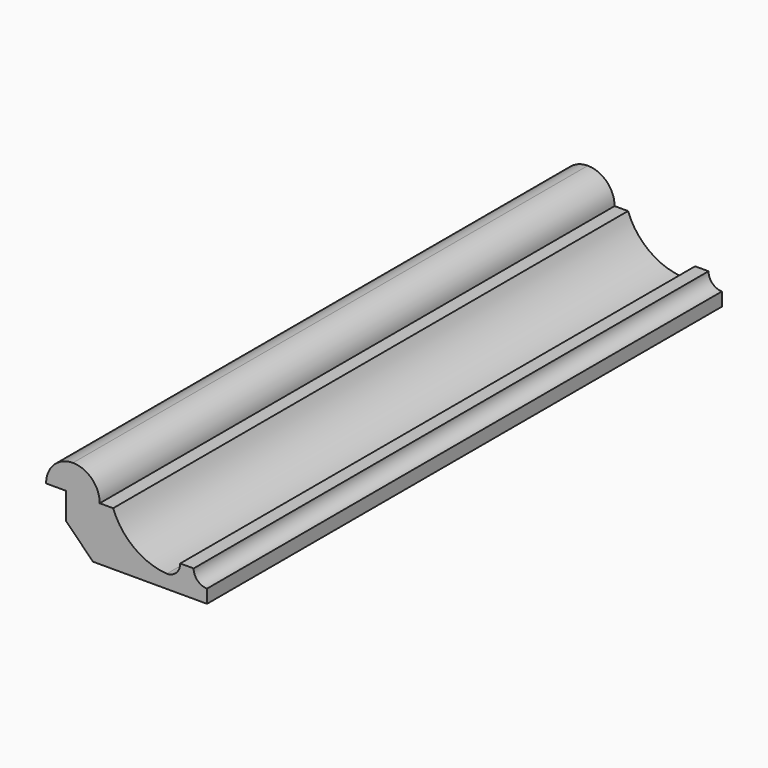
from build123d import *

# Parameters (mm, degrees)
F1_DEPTH = 152.4


# Not quite as in the source:
# - ends of sketch curves that miss each other by under 0.0002 mm in the source are joined


with BuildPart() as f1:
    # F0 (on Front) → F1 (new body)
    with BuildSketch(Plane.XZ):
        with BuildLine():
            ThreePointArc((-6.352921, 3.1764732), (-8.2136484806, 7.6686667194), (-12.705842, 9.5293942))
            ThreePointArc((-12.705842, 9.5293942), (-17.1980355194, 7.6686667194), (-19.058763, 3.1764732))
            Line((-19.058763, 3.1764732), (-14.2940786, 3.1764732))
            Line((-14.2940786, 3.1764732), (-14.2940786, -3.1764478))
            Line((-14.2940786, -3.1764478), (-7.9411576, -9.5293942))
            Line((-7.9411576, -9.5293942), (19.058763, -9.5293942))
            Line((19.058763, -9.5293942), (19.058763, -6.352921))
            ThreePointArc((19.058763, -6.352921), (16.81265726, -5.42255354), (15.8822898, -3.1764478))
            Line((15.8822898, -3.1764478), (12.705842, -3.1764478))
            ThreePointArc((12.705842, -3.1764478), (11.77549994, -5.42255354), (9.5293942, -6.352921))
            ThreePointArc((9.5293942, -6.352921), (1.7744943071, -3.4575238304), (-3.1764521069, 3.1764716036))
            Line((-3.1764521069, 3.1764716036), (-6.352921, 3.1764732))
        make_face()
    extrude(amount=F1_DEPTH)


solid = f1.part
